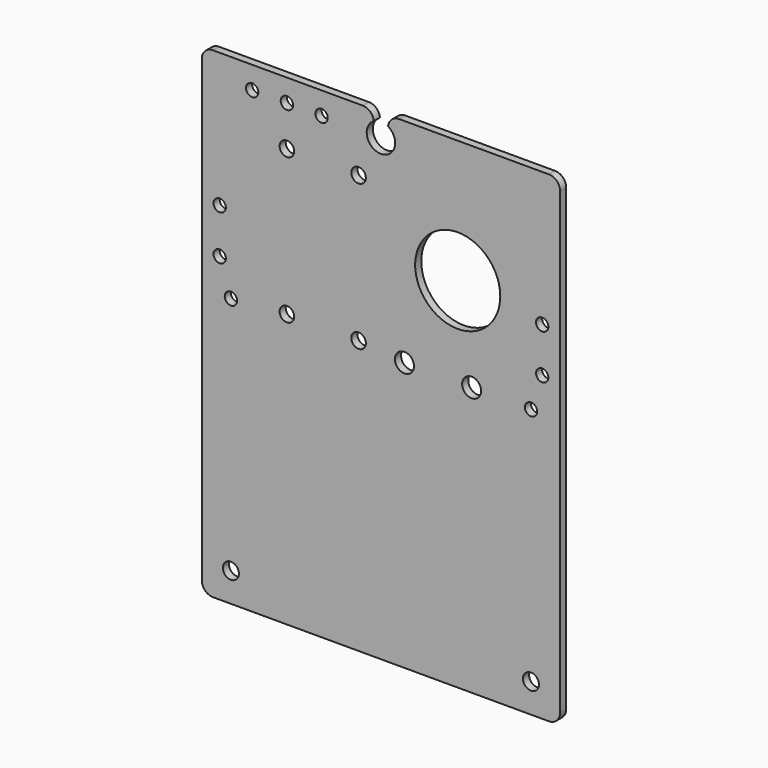
from build123d import *

# Parameters (mm, degrees)
F0_R        = 19
F1_DEPTH    = 3.42
F2_T1_DEPTH = 28.42
F2_T3_DEPTH = 28.2950568544
F4_D        = 6.5
F5_D        = 5.5
F6_D        = 8.5
F7_D        = 7.14
F8_R        = 4.5
F9_DEPTH    = 5.5
F10_D       = 4.1
F10_DEPTH   = 2.081


# Not quite as in the source:
# - a fillet or chamfer that OpenCascade refuses, or shapes differently, is made with other operations: its cross-section is extruded or revolved along the edge and cut away or added
# - a feature names something its author has since deleted; it is built from what else it names


with BuildPart() as f1:
    # F0 (on Front) → F1 (new body)
    with BuildSketch(Plane.XZ):
        with BuildLine():
            Line((-80, -107.5), (80, -107.5))
            Line((80, -107.5), (80, 107.5))
            Line((80, 107.5), (3.175, 107.5))
            Line((3.175, 107.5), (3.175, 102.999261314))
            ThreePointArc((3.175, 102.999261314), (0, 91.15), (-3.175, 102.999261314))
            Line((-3.175, 102.999261314), (-3.175, 107.5))
            Line((-3.175, 107.5), (-80, 107.5))
            Line((-80, 107.5), (-80, -107.5))
        make_face()
        with Locations((34.285, 52.5)):
            Circle(F0_R, mode=Mode.SUBTRACT)
    extrude(amount=F1_DEPTH)

    # F2: fillet of radius 5 on 6 edges, made by hand

    # F2_s2 → F2_t1 (cut)
    with BuildSketch(Plane.XZ.offset(-12.5)):
        with BuildLine():
            ThreePointArc((-75, 107.5), (-78.5355339059, 106.0355339059), (-80, 102.5))
            Line((-80, 102.5), (-80, 107.5))
            Line((-80, 107.5), (-75, 107.5))
        make_face()
        with BuildLine():
            ThreePointArc((75, -107.5), (78.5355339059, -106.0355339059), (80, -102.5))
            Line((80, -102.5), (80, -107.5))
            Line((80, -107.5), (75, -107.5))
        make_face()
        with BuildLine():
            ThreePointArc((-80, -102.5), (-78.5355339059, -106.0355339059), (-75, -107.5))
            Line((-75, -107.5), (-80, -107.5))
            Line((-80, -107.5), (-80, -102.5))
        make_face()
        with BuildLine():
            ThreePointArc((80, 102.5), (78.5355339059, 106.0355339059), (75, 107.5))
            Line((75, 107.5), (80, 107.5))
            Line((80, 107.5), (80, 102.5))
        make_face()
    extrude(amount=F2_T1_DEPTH, mode=Mode.SUBTRACT)

    # F2_s4 → F2_t3 (cut)
    with BuildSketch(Plane.XZ.offset(-12.4375284272)):
        with BuildLine():
            ThreePointArc((-8.1500113709, 107.5), (-4.7956341239, 106.2078502242), (-3.175, 102.999261314))
            Line((-3.175, 102.999261314), (-3.175, 107.5))
            Line((-3.175, 107.5), (-8.1500113709, 107.5))
        make_face()
        with BuildLine():
            ThreePointArc((8.1500113709, 107.5), (4.7956341239, 106.2078502242), (3.175, 102.999261314))
            Line((3.175, 102.999261314), (3.175, 107.5))
            Line((3.175, 107.5), (8.1500113709, 107.5))
        make_face()
    extrude(amount=F2_T3_DEPTH, mode=Mode.SUBTRACT)

    # F4 (through all)
    with Locations(Plane.XZ.offset(3.42)):
        with Locations((-42, 79.5), (-10, 79.5), (-42, 14.5), (-10, 14.5)):
            Hole(F4_D / 2)

    # F5 (through all)
    with Locations(Plane.XZ.offset(3.42)):
        with Locations((-72, 47.5), (-72, 27.5), (72, 47.5), (72, 27.5), (-57.5, 97.5), (-26.5, 97.5), (-67, 12.5), (67, 12.5), (-42, 97.5)):
            Hole(F5_D / 2)

    # F6 (through all)
    with Locations(Plane.XZ.offset(3.42)):
        with Locations((10.5, 12.5), (40.5, 12.5)):
            Hole(F6_D / 2)

    # F7 (through all)
    with Locations(Plane.XZ.offset(3.42)):
        with Locations((-67, -94.5), (67, -94.5)):
            Hole(F7_D / 2)

    # F8 (on face) → F9 (join)
    with BuildSketch(Plane.XZ.offset(3.42)):
        with Locations((10.5, 76.07)):
            Circle(F8_R)
        with Locations((58.07, 76.07)):
            Circle(F8_R)
        with Locations((58.07, 28.93)):
            Circle(F8_R)
        with Locations((10.5, 28.93)):
            Circle(F8_R)
    extrude(amount=-F9_DEPTH)

    # F10 (through all, one way)
    with BuildSketch(Plane.XZ):
        with Locations((10.5, 76.07), (58.07, 76.07), (10.5, 28.93), (58.07, 28.93)):
            Circle(F10_D / 2)
    extrude(amount=-F10_DEPTH, mode=Mode.SUBTRACT)


solid = f1.part
